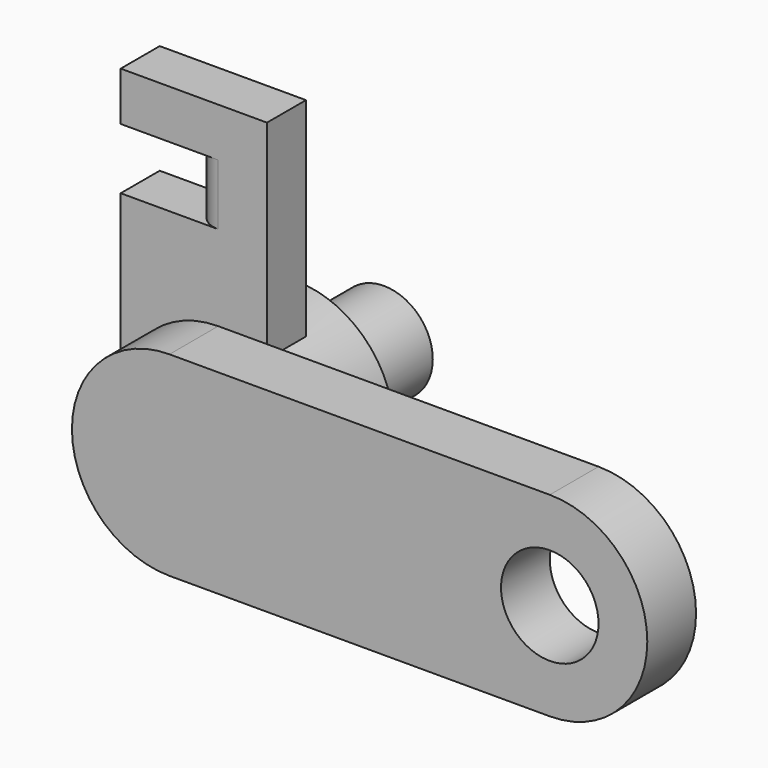
from build123d import *

# Parameters (mm, degrees)
F0_R     = 2
F1_DEPTH = 2.5
F2_DEPTH = 4
F3_DEPTH = 8.5
F4_DEPTH = 2
F5_R     = 0.99999


# Not quite as in the source:
# - a fillet or chamfer is up to 0.001 mm smaller than in the source, because OpenCascade refuses the exact size


with BuildPart() as f1:
    # F0 (on Front) → F1 (new body)
    with BuildSketch(Plane.XZ):
        with BuildLine():
            Line((2, 3.4641016151), (2, 0))
            ThreePointArc((2, 0), (0, -2), (-2, 0))
            Line((-2, 0), (-4, 0))
            ThreePointArc((-4, 0), (-2.8284271247, -2.8284271247), (0, -4))
            ThreePointArc((0, -4), (2.8284271247, -2.8284271247), (4, 0))
            ThreePointArc((4, 0), (3.4641016151, 2), (2, 3.4641016151))
        make_face()
        with BuildLine():
            ThreePointArc((0, 4), (1.0352761804, 3.8637033052), (2, 3.4641016151))
            Line((2, 3.4641016151), (2, 4))
            Line((2, 4), (0, 4))
        make_face()
        with BuildLine():
            Line((2, 4), (2, 3.4641016151))
            ThreePointArc((2, 3.4641016151), (3.4641016151, 2), (4, 0))
            ThreePointArc((4, 0), (2.8284271247, -2.8284271247), (0, -4))
            Line((0, -4), (15.6, -4))
            ThreePointArc((15.6, -4), (19.6, 0), (15.6, 4))
            Line((15.6, 4), (2, 4))
        make_face()
        with Locations((15.6, 0)):
            Circle(F0_R, mode=Mode.SUBTRACT)
        with BuildLine():
            ThreePointArc((-2, 0), (0, 2), (2, 0))
            Line((2, 0), (2, 3.4641016151))
            ThreePointArc((2, 3.4641016151), (1.0352761804, 3.8637033052), (0, 4))
            ThreePointArc((0, 4), (-2.8284271247, 2.8284271247), (-4, 0))
            Line((-4, 0), (-2, 0))
        make_face()
        with BuildLine():
            ThreePointArc((-2, 0), (0, -2), (2, 0))
            Line((2, 0), (-2, 0))
        make_face()
        with BuildLine():
            Line((-2, 0), (2, 0))
            ThreePointArc((2, 0), (0, 2), (-2, 0))
        make_face()
    extrude(amount=F1_DEPTH)

    # F0 (on Front) → F2 (join)
    with BuildSketch(Plane.XZ):
        with BuildLine():
            ThreePointArc((-2, 0), (0, 2), (2, 0))
            Line((2, 0), (2, 3.4641016151))
            ThreePointArc((2, 3.4641016151), (1.0352761804, 3.8637033052), (0, 4))
            ThreePointArc((0, 4), (-2.8284271247, 2.8284271247), (-4, 0))
            Line((-4, 0), (-2, 0))
        make_face()
        with BuildLine():
            Line((2, 3.4641016151), (2, 0))
            ThreePointArc((2, 0), (0, -2), (-2, 0))
            Line((-2, 0), (-4, 0))
            ThreePointArc((-4, 0), (-2.8284271247, -2.8284271247), (0, -4))
            ThreePointArc((0, -4), (2.8284271247, -2.8284271247), (4, 0))
            ThreePointArc((4, 0), (3.4641016151, 2), (2, 3.4641016151))
        make_face()
    extrude(amount=-F2_DEPTH)

    # F0 (on Front) → F3 (join)
    with BuildSketch(Plane.XZ):
        with BuildLine():
            ThreePointArc((-2, 0), (0, -2), (2, 0))
            Line((2, 0), (-2, 0))
        make_face()
        with BuildLine():
            Line((-2, 0), (2, 0))
            ThreePointArc((2, 0), (0, 2), (-2, 0))
        make_face()
    extrude(amount=-F3_DEPTH)

    # F0 (on Front) → F4 (join)
    with BuildSketch(Plane.XZ):
        with BuildLine():
            Line((-4, 7.5), (-4, 0))
            ThreePointArc((-4, 0), (-2.8284271247, 2.8284271247), (0, 4))
            Line((0, 4), (2, 4))
            Line((2, 4), (2, 12))
            Line((2, 12), (-4, 12))
            Line((-4, 12), (-4, 10))
            Line((-4, 10), (-1, 10))
            Line((-1, 10), (-1, 7.5))
            Line((-1, 7.5), (-4, 7.5))
        make_face()
        with BuildLine():
            ThreePointArc((0, 4), (1.0352761804, 3.8637033052), (2, 3.4641016151))
            Line((2, 3.4641016151), (2, 4))
            Line((2, 4), (0, 4))
        make_face()
        with BuildLine():
            ThreePointArc((-2, 0), (0, 2), (2, 0))
            Line((2, 0), (2, 3.4641016151))
            ThreePointArc((2, 3.4641016151), (1.0352761804, 3.8637033052), (0, 4))
            ThreePointArc((0, 4), (-2.8284271247, 2.8284271247), (-4, 0))
            Line((-4, 0), (-2, 0))
        make_face()
        with BuildLine():
            ThreePointArc((-2, 0), (0, -2), (2, 0))
            Line((2, 0), (-2, 0))
        make_face()
        with BuildLine():
            Line((-2, 0), (2, 0))
            ThreePointArc((2, 0), (0, 2), (-2, 0))
        make_face()
        with BuildLine():
            Line((2, 3.4641016151), (2, 0))
            ThreePointArc((2, 0), (0, -2), (-2, 0))
            Line((-2, 0), (-4, 0))
            ThreePointArc((-4, 0), (-2.8284271247, -2.8284271247), (0, -4))
            ThreePointArc((0, -4), (2.8284271247, -2.8284271247), (4, 0))
            ThreePointArc((4, 0), (3.4641016151, 2), (2, 3.4641016151))
        make_face()
    extrude(amount=-F4_DEPTH)

    # F5 (radius 1 in the source; OpenCascade refuses exactly that, so slightly less here)
    f5_edges = [f1.edges().sort_by_distance(p)[0] for p in [
        (-1, 0, 8.75),
        (-1, 2, 8.75),
    ]]
    fillet(f5_edges, radius=F5_R)


solid = f1.part
